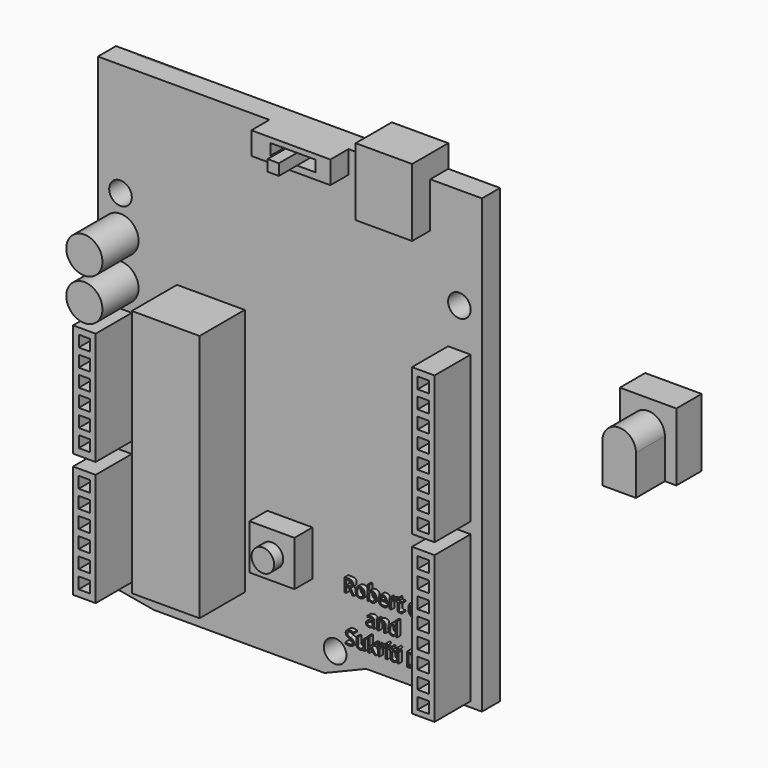
from build123d import *

# Parameters (mm, degrees)
F0_R          = 1.5875
F0_W          = 3.175
F0_H          = 15.875
F0_W_2        = 6.35
F0_H_2        = 6.35
F0_W_3        = 9.525
F0_H_3        = 34.925
F0_H_4        = 20.6375
F0_R_2        = 2.54
F0_W_4        = 7.9502
F0_H_5        = 9.525
F2_DEPTH      = 3.175
F0_W_5        = 11.1125
F0_H_6        = 3.175
F3_DEPTH      = 6.35
F0_W_6        = 1.5875
F0_H_7        = 1.570019871
F4_DEPTH      = 9.525
F0_W_7        = 1.6002
F0_H_8        = 1.6002
F0_H_9        = 1.5911653172
F0_H_10       = 1.5924457857
F0_H_11       = 1.5955853742
F0_H_12       = 1.5875
F0_H_13       = 1.6087964177
F0_H_14       = 1.588659361
F0_H_15       = 1.6127470881
F5_DEPTH      = 9.525
F6_DEPTH      = 11.1125
F0_W_8        = 7.9375
F7_DEPTH      = 6.35
F8_DEPTH      = 6.35
F9_DEPTH      = 7.9375
F11_DEPTH     = 0.254
F10_TEXT_SIZE = 2.6458333333
F12_DEPTH     = 3.81
F13_DEPTH     = 4.445
F1_R          = 0.396875
F1_R_2        = 0.79375
F14_DEPTH     = 9.525
F15_DEPTH     = 0.0254
F16_DEPTH     = 0.0254
F17_DEPTH     = 0.0254
F0_W_9        = 2.620653346
F0_W_10       = 2.141846654
F18_DEPTH     = 0.0254
F19_DEPTH     = 0.0254
F20_DEPTH     = 9.525


# Not quite as in the source:
# - Text() gives the source's letters only with a copy of the font that has no kerning and outlines rounded to 1/6400 em; it was checked with that copy


with BuildPart() as f2:
    # F0 (on Front) → F2 (new body)
    with BuildSketch(Plane.XZ):
        Polygon((-32.1187235904, 35.3362501681), (-35.2937235904, 35.3362501681), (-35.2937235904, -29.7512498319), (-32.1187235904, -29.7512498319), (-27.4279320389, -30.5745850433), (-3.4351130193, -30.5745850433), (0.9799254118, -28.7552525581), (2.4193077689, -28.1621172725), (18.6812764096, -28.1621172725), (18.6812764096, 35.3362501681), (11.4064374939, 35.3362501681), (11.4064374939, 28.9862501681), (3.4689374939, 28.9862501681), (3.4689374939, 35.3362501681), (-0.0808204204, 35.3362501681), (-0.0808204204, 32.1612501681), (-11.1933204204, 32.1612501681), (-11.1933204204, 35.3362501681), (-24.1685235904, 35.3362501681), (-24.1685235904, 25.8112501681), (-32.1187235904, 25.8112501681), align=None)
        with Locations((-27.7165417003, -27.3868850433)):
            Circle(F0_R, mode=Mode.SUBTRACT)
        with Locations((-32.1187235904, -20.2262498319)):
            Rectangle(F0_W, F0_H, mode=Mode.SUBTRACT)
        with Locations((-8.3062235904, -16.2870850433)):
            Rectangle(F0_W_2, F0_H_2, mode=Mode.SUBTRACT)
        with Locations((-32.1187235904, -2.7637498319)):
            Rectangle(F0_W, F0_H, mode=Mode.SUBTRACT)
        with Locations((-19.4187235904, -6.7620850433)):
            Rectangle(F0_W_3, F0_H_3, mode=Mode.SUBTRACT)
        with Locations((-1.9562235904, -27.3995850433)):
            Circle(F0_R, mode=Mode.SUBTRACT)
        with Locations((15.5062764096, -17.0496172725)):
            Rectangle(F0_W, F0_H_4, mode=Mode.SUBTRACT)
        with Locations((-32.1187235904, 8.5075001681)):
            Circle(F0_R_2, mode=Mode.SUBTRACT)
        with Locations((-32.1187235904, 14.3812501681)):
            Circle(F0_R_2, mode=Mode.SUBTRACT)
        with Locations((-32.1187235904, 19.4612501681)):
            Circle(F0_R, mode=Mode.SUBTRACT)
        with Locations((15.5062764096, 5.1753827275)):
            Rectangle(F0_W, F0_H_4, mode=Mode.SUBTRACT)
        with Locations((15.5062764096, 21.0487501681)):
            Circle(F0_R, mode=Mode.SUBTRACT)
        with Locations((-28.1436235904, 30.5737501681)):
            Rectangle(F0_W_4, F0_H_5)
    extrude(amount=F2_DEPTH)

    # F0 (on Front) → F3 (join)
    with BuildSketch(Plane.XZ):
        with Locations((-5.6370704204, 33.7487501681)):
            Rectangle(F0_W_5, F0_H_6)
        Polygon((-6.3664172776, 33.0660454929), (-8.5082639316, 33.0660454929), (-8.5082639316, 34.6360653639), (-6.3664172776, 34.6360653639), (-4.7789172776, 34.6360653639), (-2.1582639316, 34.6360653639), (-2.1582639316, 33.0660454929), (-4.7789172776, 33.0660454929), align=None, mode=Mode.SUBTRACT)
    extrude(amount=F3_DEPTH)

    # F0 (on Front) → F4 (join)
    with BuildSketch(Plane.XZ):
        with Locations((-5.5726672776, 33.8510554284)):
            Rectangle(F0_W_6, F0_H_7)
    extrude(amount=F4_DEPTH)

    # F0 (on Front) → F5 (join)
    with BuildSketch(Plane.XZ):
        with Locations((15.5062764096, -17.0496172725)):
            Rectangle(F0_W, F0_H_4)
        with Locations((15.5062764096, -25.8443672725)):
            Rectangle(F0_W_7, F0_H_8, mode=Mode.SUBTRACT)
        with Locations((15.5062764096, -23.3551672725)):
            Rectangle(F0_W_7, F0_H_8, mode=Mode.SUBTRACT)
        with Locations((15.5062764096, -20.8659672725)):
            Rectangle(F0_W_7, F0_H_8, mode=Mode.SUBTRACT)
        with Locations((15.5062764096, -18.3767672725)):
            Rectangle(F0_W_7, F0_H_8, mode=Mode.SUBTRACT)
        with Locations((15.5062764096, -15.8875672725)):
            Rectangle(F0_W_7, F0_H_8, mode=Mode.SUBTRACT)
        with Locations((15.5062764096, -13.3983672725)):
            Rectangle(F0_W_7, F0_H_8, mode=Mode.SUBTRACT)
        with Locations((15.5062764096, -10.9091672725)):
            Rectangle(F0_W_7, F0_H_8, mode=Mode.SUBTRACT)
        with Locations((15.5062764096, -8.4199672725)):
            Rectangle(F0_W_7, F0_H_8, mode=Mode.SUBTRACT)
        with Locations((15.5062764096, 5.1753827275)):
            Rectangle(F0_W, F0_H_4)
        with Locations((15.5062764096, -3.602481091)):
            Rectangle(F0_W_7, F0_H_9, mode=Mode.SUBTRACT)
        with Locations((15.5062764096, -1.1216755395)):
            Rectangle(F0_W_7, F0_H_10, mode=Mode.SUBTRACT)
        with Locations((15.5062764096, 1.3636473533)):
            Rectangle(F0_W_7, F0_H_8, mode=Mode.SUBTRACT)
        with Locations((15.5062764096, 3.8505400404)):
            Rectangle(F0_W_7, F0_H_11, mode=Mode.SUBTRACT)
        with Locations((15.5062764096, 6.3374327275)):
            Rectangle(F0_W_7, F0_H_8, mode=Mode.SUBTRACT)
        with Locations((15.5062764096, 8.8266327275)):
            Rectangle(F0_W_7, F0_H_8, mode=Mode.SUBTRACT)
        with Locations((15.5062764096, 11.3158327275)):
            Rectangle(F0_W_7, F0_H_8, mode=Mode.SUBTRACT)
        with Locations((15.5062764096, 13.8050327275)):
            Rectangle(F0_W_7, F0_H_8, mode=Mode.SUBTRACT)
        with Locations((-32.1187235904, -2.7637498319)):
            Rectangle(F0_W, F0_H)
        with Locations((-32.1123735904, -8.9486498319)):
            Rectangle(F0_W_6, F0_H_8, mode=Mode.SUBTRACT)
        with Locations((-32.1123735904, -6.4594498319)):
            Rectangle(F0_W_6, F0_H_8, mode=Mode.SUBTRACT)
        with Locations((-32.1123735904, -3.9702498319)):
            Rectangle(F0_W_6, F0_H_8, mode=Mode.SUBTRACT)
        with Locations((-32.1123735904, -1.4810498319)):
            Rectangle(F0_W_6, F0_H_8, mode=Mode.SUBTRACT)
        Polygon((-32.9061235904, 1.2243902311), (-32.9061235904, 1.2507905485), (-32.9061235904, 1.8082501681), (-31.3186235904, 1.8082501681), (-31.3186235904, 0.2080501681), (-32.9061235904, 0.2080501681), align=None, mode=Mode.SUBTRACT)
        with Locations((-32.1123735904, 3.4910001681)):
            Rectangle(F0_W_6, F0_H_12, mode=Mode.SUBTRACT)
        with Locations((-32.1187235904, -20.2262498319)):
            Rectangle(F0_W, F0_H)
        with Locations((-32.1187235904, -26.4291544899)):
            Rectangle(F0_W_7, F0_H_13, mode=Mode.SUBTRACT)
        with Locations((-32.1187235904, -23.9414266005)):
            Rectangle(F0_W_7, F0_H_14, mode=Mode.SUBTRACT)
        with Locations((-32.1187235904, -21.45799692)):
            Rectangle(F0_W_7, F0_H_8, mode=Mode.SUBTRACT)
        with Locations((-32.1187235904, -18.962523376)):
            Rectangle(F0_W_7, F0_H_15, mode=Mode.SUBTRACT)
        with Locations((-32.1187235904, -16.4670498319)):
            Rectangle(F0_W_7, F0_H_8, mode=Mode.SUBTRACT)
        with Locations((-32.1187235904, -13.9778498319)):
            Rectangle(F0_W_7, F0_H_8, mode=Mode.SUBTRACT)
    extrude(amount=F5_DEPTH)

    # F0 (on Front) → F6 (join)
    with BuildSketch(Plane.XZ):
        with Locations((-19.4187235904, -6.7620850433)):
            Rectangle(F0_W_3, F0_H_3)
    extrude(amount=F6_DEPTH)

    # F0 (on Front) → F7 (join)
    with BuildSketch(Plane.XZ):
        Polygon((3.4689374939, 36.5110784769), (3.4689374939, 35.3362501681), (11.4064374939, 35.3362501681), (11.4064374939, 36.5110784769), (11.4064374939, 38.5112501681), (11.1429411918, 38.5112501681), (3.7291275803, 38.5112501681), (3.4689374939, 38.5112501681), align=None)
        with Locations((7.4376874939, 32.1612501681)):
            Rectangle(F0_W_8, F0_H_2)
    extrude(amount=F7_DEPTH)

    # F0 (on Front) → F8 (join)
    with BuildSketch(Plane.XZ):
        with Locations((-8.3062235904, -16.2870850433)):
            Rectangle(F0_W_2, F0_H_2)
        with Locations((-8.3062235904, -16.2854524838)):
            Circle(F0_R, mode=Mode.SUBTRACT)
    extrude(amount=F8_DEPTH)

    # F0 (on Front) → F9 (join)
    with BuildSketch(Plane.XZ):
        with Locations((-8.3062235904, -16.2854524838)):
            Circle(F0_R)
    extrude(amount=F9_DEPTH)

    # F0 (on Front) → F15 (join)
    with BuildSketch(Plane.XZ):
        with Locations((-32.1123735904, -1.4810498319)):
            Rectangle(F0_W_6, F0_H_8)
        Polygon((-32.9061235904, 1.8082501681), (-32.9061235904, 1.2507905485), (-32.9061235904, 1.2243902311), (-32.9061235904, 0.2080501681), (-31.3186235904, 0.2080501681), (-31.3186235904, 1.8082501681), align=None)
        with Locations((-32.1123735904, 3.4910001681)):
            Rectangle(F0_W_6, F0_H_12)
        with Locations((-32.1123735904, -3.9702498319)):
            Rectangle(F0_W_6, F0_H_8)
        with Locations((-32.1123735904, -8.9486498319)):
            Rectangle(F0_W_6, F0_H_8)
        with Locations((-32.1123735904, -6.4594498319)):
            Rectangle(F0_W_6, F0_H_8)
    extrude(amount=F15_DEPTH)

    # F0 (on Front) → F16 (join)
    with BuildSketch(Plane.XZ):
        with Locations((-32.1187235904, -13.9778498319)):
            Rectangle(F0_W_7, F0_H_8)
        with Locations((-32.1187235904, -16.4670498319)):
            Rectangle(F0_W_7, F0_H_8)
        with Locations((-32.1187235904, -18.962523376)):
            Rectangle(F0_W_7, F0_H_15)
        with Locations((-32.1187235904, -21.45799692)):
            Rectangle(F0_W_7, F0_H_8)
        with Locations((-32.1187235904, -23.9414266005)):
            Rectangle(F0_W_7, F0_H_14)
        with Locations((-32.1187235904, -26.4291544899)):
            Rectangle(F0_W_7, F0_H_13)
    extrude(amount=F16_DEPTH)

    # F0 (on Front) → F17 (join)
    with BuildSketch(Plane.XZ):
        with Locations((15.5062764096, 13.8050327275)):
            Rectangle(F0_W_7, F0_H_8)
        with Locations((15.5062764096, -1.1216755395)):
            Rectangle(F0_W_7, F0_H_10)
        with Locations((15.5062764096, 1.3636473533)):
            Rectangle(F0_W_7, F0_H_8)
        with Locations((15.5062764096, 3.8505400404)):
            Rectangle(F0_W_7, F0_H_11)
        with Locations((15.5062764096, 6.3374327275)):
            Rectangle(F0_W_7, F0_H_8)
        with Locations((15.5062764096, 8.8266327275)):
            Rectangle(F0_W_7, F0_H_8)
        with Locations((15.5062764096, 11.3158327275)):
            Rectangle(F0_W_7, F0_H_8)
        with Locations((15.5062764096, -3.602481091)):
            Rectangle(F0_W_7, F0_H_9)
    extrude(amount=F17_DEPTH)

    # F0 (on Front) → F18 (join)
    with BuildSketch(Plane.XZ):
        with Locations((-3.4685906046, 33.8510554284)):
            Rectangle(F0_W_9, F0_H_7)
        with Locations((-7.4373406046, 33.8510554284)):
            Rectangle(F0_W_10, F0_H_7)
    extrude(amount=F18_DEPTH)

    # F0 (on Front) → F19 (join)
    with BuildSketch(Plane.XZ):
        with Locations((15.5062764096, -13.3983672725)):
            Rectangle(F0_W_7, F0_H_8)
        with Locations((15.5062764096, -18.3767672725)):
            Rectangle(F0_W_7, F0_H_8)
        with Locations((15.5062764096, -15.8875672725)):
            Rectangle(F0_W_7, F0_H_8)
        with Locations((15.5062764096, -20.8659672725)):
            Rectangle(F0_W_7, F0_H_8)
        with Locations((15.5062764096, -23.3551672725)):
            Rectangle(F0_W_7, F0_H_8)
        with Locations((15.5062764096, -25.8443672725)):
            Rectangle(F0_W_7, F0_H_8)
        with Locations((15.5062764096, -10.9091672725)):
            Rectangle(F0_W_7, F0_H_8)
        with Locations((15.5062764096, -8.4199672725)):
            Rectangle(F0_W_7, F0_H_8)
    extrude(amount=F19_DEPTH)

    # F0 (on Front) → F20 (join)
    with BuildSketch(Plane.XZ):
        with Locations((-32.1187235904, 14.3812501681)):
            Circle(F0_R_2)
        with Locations((-32.1187235904, 8.5075001681)):
            Circle(F0_R_2)
    extrude(amount=F20_DEPTH)


with BuildPart() as f11:
    # F0 (on Front) → F11 (new body)
    with BuildSketch(Plane.XZ):
        with Locations((-28.1436235904, 30.5737501681)):
            Rectangle(F0_W_4, F0_H_5)
    extrude(amount=F11_DEPTH)


with BuildPart() as f12:
    # F10 (on Front) → F12 (new body)
    with BuildSketch(Plane.XZ):
        with Locations((-0.373039606, -19.2721172725)):
            Text('Robert G', F10_TEXT_SIZE, font='Open Sans', text_align=(TextAlign.LEFT, TextAlign.BOTTOM))
        with Locations((2.7693008888, -22.4471172725)):
            Text('and', F10_TEXT_SIZE, font='Open Sans', text_align=(TextAlign.LEFT, TextAlign.BOTTOM))
        with Locations((-0.1223055565, -25.6221172725)):
            Text('Sukriti D', F10_TEXT_SIZE, font='Open Sans', text_align=(TextAlign.LEFT, TextAlign.BOTTOM))
    extrude(amount=F12_DEPTH)


with BuildPart() as f13:
    # F1 (on Front) → F13 (new body)
    with BuildSketch(Plane.XZ):
        with BuildLine():
            Line((47.0150679946, 19.0736745853), (39.0775679946, 19.0736745853))
            Line((39.0775679946, 19.0736745853), (39.0775679946, 9.5486745853))
            Line((39.0775679946, 9.5486745853), (40.6914339429, 9.5486745853))
            Line((40.6914339429, 9.5486745853), (40.6914339429, 15.1312905336))
            ThreePointArc((40.6914339429, 15.1312905336), (43.0463179946, 17.4861745853), (45.4012020463, 15.1312905336))
            Line((45.4012020463, 15.1312905336), (45.4012020463, 9.5486745853))
            Line((45.4012020463, 9.5486745853), (47.0150679946, 9.5486745853))
            Line((47.0150679946, 9.5486745853), (47.0150679946, 19.0736745853))
        make_face()
        with BuildLine():
            Line((40.6914339429, 15.1312905336), (40.6914339429, 9.5486745853))
            Line((40.6914339429, 9.5486745853), (45.4012020463, 9.5486745853))
            Line((45.4012020463, 9.5486745853), (45.4012020463, 15.1312905336))
            ThreePointArc((45.4012020463, 15.1312905336), (44.7300116448, 13.484883965), (43.0990465859, 12.7769968831))
            ThreePointArc((43.0990465859, 12.7769968831), (43.0726839429, 12.7765540868), (43.0463179946, 12.7764064819))
            ThreePointArc((43.0463179946, 12.7764064819), (43.0199520463, 12.7765540868), (42.9935894033, 12.7769968831))
            ThreePointArc((42.9935894033, 12.7769968831), (41.3626243443, 13.484883965), (40.6914339429, 15.1312905336))
        make_face()
    extrude(amount=F13_DEPTH)


with BuildPart() as f13b:
    # F1 (on Front) → F13, piece 2 (new body)
    with BuildSketch(Plane.XZ):
        with Locations((43.0463179946, 15.1312905336)):
            Circle(F1_R)
    extrude(amount=F13_DEPTH)


with BuildPart() as f14:
    # F1 (on Front) → F14 (new body)
    with BuildSketch(Plane.XZ):
        with BuildLine():
            ThreePointArc((45.4012020463, 15.1312905336), (43.0463179946, 17.4861745853), (40.6914339429, 15.1312905336))
            ThreePointArc((40.6914339429, 15.1312905336), (41.3626243443, 13.484883965), (42.9935894033, 12.7769968831))
            ThreePointArc((42.9935894033, 12.7769968831), (43.0199520463, 12.7765540868), (43.0463179946, 12.7764064819))
            ThreePointArc((43.0463179946, 12.7764064819), (43.0726839429, 12.7765540868), (43.0990465859, 12.7769968831))
            ThreePointArc((43.0990465859, 12.7769968831), (44.7300116448, 13.484883965), (45.4012020463, 15.1312905336))
        make_face()
        with Locations((43.0463179946, 15.1312905336)):
            Circle(F1_R_2, mode=Mode.SUBTRACT)
        with BuildLine():
            Line((40.6914339429, 15.1312905336), (40.6914339429, 9.5486745853))
            Line((40.6914339429, 9.5486745853), (45.4012020463, 9.5486745853))
            Line((45.4012020463, 9.5486745853), (45.4012020463, 15.1312905336))
            ThreePointArc((45.4012020463, 15.1312905336), (44.7300116448, 13.484883965), (43.0990465859, 12.7769968831))
            ThreePointArc((43.0990465859, 12.7769968831), (43.0726839429, 12.7765540868), (43.0463179946, 12.7764064819))
            ThreePointArc((43.0463179946, 12.7764064819), (43.0199520463, 12.7765540868), (42.9935894033, 12.7769968831))
            ThreePointArc((42.9935894033, 12.7769968831), (41.3626243443, 13.484883965), (40.6914339429, 15.1312905336))
        make_face()
        with Locations((43.0463179946, 15.1312905336)):
            Circle(F1_R_2)
        with Locations((43.0463179946, 15.1312905336)):
            Circle(F1_R, mode=Mode.SUBTRACT)
        with Locations((43.0463179946, 15.1312905336)):
            Circle(F1_R)
    extrude(amount=F14_DEPTH)


solid = Compound([f2.part, f11.part, f12.part, f13.part, f13b.part, f14.part])
